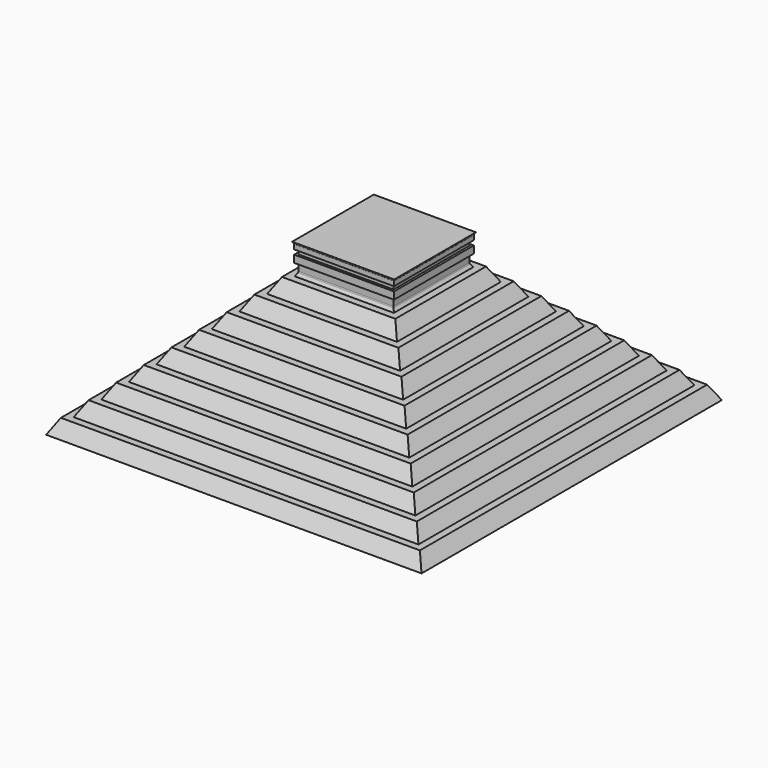
from build123d import *

# Parameters (mm, degrees)
F3_DEPTH  = 1003.8461
F4_W      = 2548.7215518951
F4_H      = 1253.2386779785
F5_DEPTH  = 1003.8461
F8_DEPTH  = 273.05
F10_DEPTH = 546.1
F12_DEPTH = 273.05


# Not quite as in the source:
# - ends of sketch curves that miss each other by under 0.0002 mm in the source are joined


with BuildPart() as f3:
    # F2 (on Front) → F3 (new body, symmetric)
    with BuildSketch(Plane.XZ):
        Polygon((-959.8512426, -348.3992524), (-1003.845338, -424.5992524), (76.2, -424.5992524), (1003.845338, -424.5992524), (959.8512426, -348.3992524), (921.7512426, -348.3992524), (877.7571472, -272.1992524), (839.6571472, -272.1992524), (795.6630772, -195.9992524), (757.5630772, -195.9992524), (713.5689818, -119.7992524), (675.4689818, -119.7992524), (631.4748864, -43.5992524), (593.3748864, -43.5992524), (549.380791, 32.6007476), (511.280791, 32.6007476), (467.2866956, 108.8007476), (429.1866956, 108.8007476), (385.1926002, 185.0007476), (347.0926002, 185.0007476), (303.0985302, 261.2007476), (264.9985302, 261.2007476), (-264.9985302, 261.2007476), (-303.0985302, 261.2007476), (-347.0926256, 185.0007476), (-385.1926256, 185.0007476), (-429.1866956, 108.8007476), (-467.2866956, 108.8007476), (-511.280791, 32.6007476), (-549.380791, 32.6007476), (-593.3748864, -43.5992524), (-631.4748864, -43.5992524), (-675.4689818, -119.7992524), (-713.5689818, -119.7992524), (-757.5630772, -195.9992524), (-795.6630772, -195.9992524), (-839.6571472, -272.1992524), (-877.7571472, -272.1992524), (-921.7512426, -348.3992524), align=None)
    extrude(amount=F3_DEPTH, both=True)

    # F4 (on Right) → F5 (cut, symmetric)
    with BuildSketch(Plane.YZ):
        with Locations((-39.1746759415, -156.0024023056)):
            Rectangle(F4_W, F4_H)
        Polygon((1003.845338, -424.5992524), (76.2, -424.5992524), (-1003.845338, -424.5992524), (-959.8512426, -348.3992524), (-921.7512426, -348.3992524), (-877.7571472, -272.1992524), (-839.6571472, -272.1992524), (-795.6630772, -195.9992524), (-757.5630772, -195.9992524), (-713.5689818, -119.7992524), (-675.4689818, -119.7992524), (-631.4748864, -43.5992524), (-593.3748864, -43.5992524), (-549.380791, 32.6007476), (-511.280791, 32.6007476), (-467.2866956, 108.8007476), (-429.1866956, 108.8007476), (-385.1926256, 185.0007476), (-347.0926256, 185.0007476), (-303.0985302, 261.2007476), (-264.9985302, 261.2007476), (264.9985302, 261.2007476), (303.0985302, 261.2007476), (347.0926002, 185.0007476), (385.1926002, 185.0007476), (429.1866956, 108.8007476), (467.2866956, 108.8007476), (511.280791, 32.6007476), (549.380791, 32.6007476), (593.3748864, -43.5992524), (631.4748864, -43.5992524), (675.4689818, -119.7992524), (713.5689818, -119.7992524), (757.5630772, -195.9992524), (795.6630772, -195.9992524), (839.6571472, -272.1992524), (877.7571472, -272.1992524), (921.7512426, -348.3992524), (959.8512426, -348.3992524), align=None, mode=Mode.SUBTRACT)
    extrude(amount=F5_DEPTH, both=True, mode=Mode.SUBTRACT)

    # F6 (on Front) → F8 (join, symmetric)
    with BuildSketch(Plane.XZ):
        Polygon((273.05, 261.2007476), (273.05, 424.5992778), (-273.05, 424.5992778), (-273.05, 261.2007476), (-264.9985302, 261.2007476), (264.9985302, 261.2007476), align=None)
    extrude(amount=F8_DEPTH, both=True)

    # F9 (on face) → F10 (cut, through all)
    with BuildSketch(Plane.YZ.offset(273.05)):
        with BuildLine():
            Line((273.05, 424.5992778), (267.5507476, 415.0742778))
            ThreePointArc((267.5507476, 415.0742778), (266.9163715798, 413.542780889), (266.7, 411.8992778))
            Line((266.7, 411.8992778), (266.7, 404.489539))
            Line((266.7, 404.489539), (266.7, 387.7583304))
            Line((266.7, 387.7583304), (254, 387.7583304))
            Line((254, 387.7583304), (254, 363.2431648))
            Line((254, 363.2431648), (266.7, 363.2431648))
            Line((266.7, 363.2431648), (266.7, 354.1319562))
            Line((266.7, 354.1319562), (266.7, 324.479539))
            Line((266.7, 324.479539), (254, 324.479539))
            Line((254, 324.479539), (254, 283.6537126))
            ThreePointArc((254, 283.6537126), (254.4327415162, 280.3667125557), (255.701475479, 277.3037158787))
            Line((255.701475479, 277.3037158787), (264.9985302, 261.2007476))
            Line((264.9985302, 261.2007476), (273.05, 261.2007476))
            Line((273.05, 261.2007476), (273.05, 424.5992778))
        make_face()
        with BuildLine():
            Line((-264.9985302, 261.2007476), (-255.7014698, 277.3037126))
            ThreePointArc((-255.7014698, 277.3037126), (-254.4327415162, 280.3667125557), (-254, 283.6537126))
            Line((-254, 283.6537126), (-254, 324.479539))
            Line((-254, 324.479539), (-266.7, 324.479539))
            Line((-266.7, 324.479539), (-266.7, 354.1319562))
            Line((-266.7, 354.1319562), (-266.7, 363.2431648))
            Line((-266.7, 363.2431648), (-254, 363.2431648))
            Line((-254, 363.2431648), (-254, 387.7583304))
            Line((-254, 387.7583304), (-266.7, 387.7583304))
            Line((-266.7, 387.7583304), (-266.7, 404.489539))
            Line((-266.7, 404.489539), (-266.7, 411.8992778))
            ThreePointArc((-266.7, 411.8992778), (-266.9163715798, 413.542780889), (-267.5507409145, 415.0742816599))
            Line((-267.5507409145, 415.0742816599), (-273.05, 424.5992778))
            Line((-273.05, 424.5992778), (-273.05, 261.2007476))
            Line((-273.05, 261.2007476), (-264.9985302, 261.2007476))
        make_face()
    extrude(amount=-F10_DEPTH, mode=Mode.SUBTRACT)

    # F11 (on Front) → F12 (cut, symmetric)
    with BuildSketch(Plane.XZ):
        with BuildLine():
            ThreePointArc((254, 283.6537126), (254.4327415162, 280.3667125557), (255.701475479, 277.3037158787))
            Line((255.701475479, 277.3037158787), (264.9985302, 261.2007476))
            Line((264.9985302, 261.2007476), (273.05, 261.2007476))
            Line((273.05, 261.2007476), (273.05, 424.5992778))
            Line((273.05, 424.5992778), (267.5507476, 415.0742778))
            ThreePointArc((267.5507476, 415.0742778), (266.9163715798, 413.542780889), (266.7, 411.8992778))
            Line((266.7, 411.8992778), (266.7, 404.489539))
            Line((266.7, 404.489539), (266.7, 387.7583304))
            Line((266.7, 387.7583304), (254, 387.7583304))
            Line((254, 387.7583304), (254, 363.2431648))
            Line((254, 363.2431648), (266.7, 363.2431648))
            Line((266.7, 363.2431648), (266.7, 354.1319562))
            Line((266.7, 354.1319562), (266.7, 324.479539))
            Line((266.7, 324.479539), (254, 324.479539))
            Line((254, 324.479539), (254, 283.6537126))
        make_face()
        with BuildLine():
            ThreePointArc((-266.7, 411.8992778), (-266.9163715798, 413.542780889), (-267.5507409145, 415.0742816599))
            Line((-267.5507409145, 415.0742816599), (-273.05, 424.5992778))
            Line((-273.05, 424.5992778), (-273.05, 261.2007476))
            Line((-273.05, 261.2007476), (-264.9985302, 261.2007476))
            Line((-264.9985302, 261.2007476), (-255.7014698, 277.3037126))
            ThreePointArc((-255.7014698, 277.3037126), (-254.4327415162, 280.3667125557), (-254, 283.6537126))
            Line((-254, 283.6537126), (-254, 324.479539))
            Line((-254, 324.479539), (-266.7, 324.479539))
            Line((-266.7, 324.479539), (-266.7, 354.1319562))
            Line((-266.7, 354.1319562), (-266.7, 363.2431648))
            Line((-266.7, 363.2431648), (-254, 363.2431648))
            Line((-254, 363.2431648), (-254, 387.7583304))
            Line((-254, 387.7583304), (-266.7, 387.7583304))
            Line((-266.7, 387.7583304), (-266.7, 404.489539))
            Line((-266.7, 404.489539), (-266.7, 411.8992778))
        make_face()
    extrude(amount=F12_DEPTH, both=True, mode=Mode.SUBTRACT)


solid = f3.part
